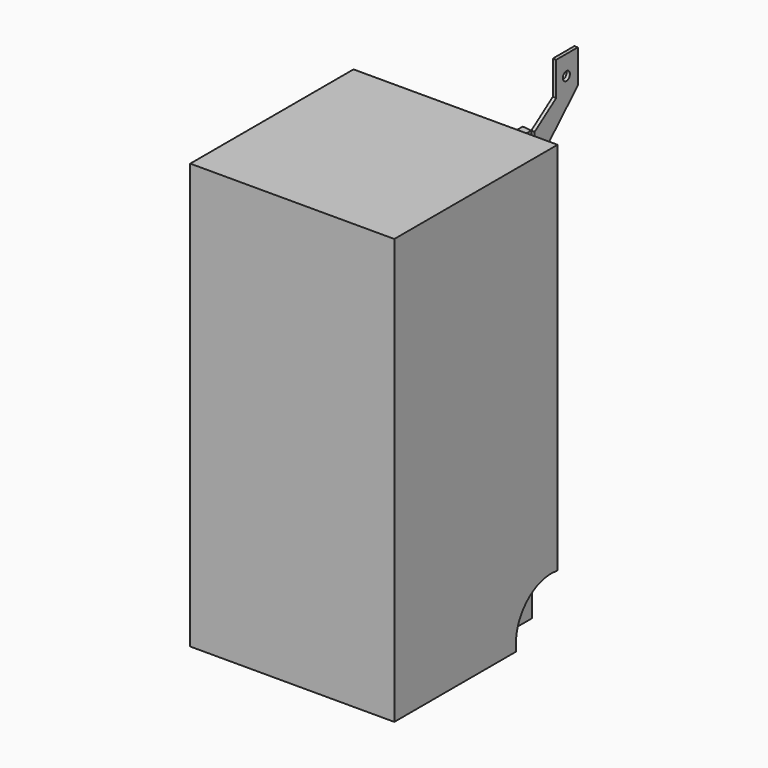
from build123d import *

# Parameters (mm, degrees)
F0_W      = 120
F0_H      = 120
F1_DEPTH  = 250
F4_DEPTH  = 15
F5_DEPTH  = 15
F6_R      = 5
F7_DEPTH  = 90
F11_DEPTH = 10
F12_R     = 2.5839894192
F13_DEPTH = 2


# Not quite as in the source:
# - the program builds the solid bodies; features that only make, move or delete a surface that nothing else refers to are left out


with BuildPart() as f1:
    # F0 (on Top) → F1 (new body)
    with BuildSketch(Plane.XY):
        with Locations((-36.543828845, 41.7243348807)):
            Rectangle(F0_W, F0_H)
    extrude(amount=F1_DEPTH)

    # F3 (on face) → F4 (cut)
    with BuildSketch(Plane(origin=(-96.543828845, 0, 0), x_dir=(0, -1, 0), z_dir=(-1, 0, 0))):
        with BuildLine():
            Line((-101.7243348807, 0), (-71.6849491, 0))
            ThreePointArc((-71.6849491, 0), (-78.6384158471, 23.222277743), (-101.7243348807, 30.6158713042))
            Line((-101.7243348807, 30.6158713042), (-101.7243348807, 0))
        make_face()
    extrude(amount=-F4_DEPTH, mode=Mode.SUBTRACT)

    # F2 (on face) → F5 (cut)
    with BuildSketch(Plane.YZ.offset(23.456171155)):
        with BuildLine():
            Line((101.7243348807, 0), (101.7243348807, 29.543299228))
            ThreePointArc((101.7243348807, 29.543299228), (78.9226920916, 22.6021851134), (71.3572967199, 0))
            Line((71.3572967199, 0), (101.7243348807, 0))
        make_face()
    extrude(amount=-F5_DEPTH, mode=Mode.SUBTRACT)

    # F6 (on face) → F7 (cut)
    with BuildSketch(Plane.YZ.offset(8.456171155)):
        with Locations((89.8642912507, 12.767852284)):
            Circle(F6_R)
    extrude(amount=-F7_DEPTH, mode=Mode.SUBTRACT)

    # F10 (on face) → F11 (join)
    with BuildSketch(Plane(origin=(0, 101.7243348807, 0), x_dir=(-1, 0, 0), z_dir=(0, 1, 0))):
        Polygon((5.0153527409, 246.1044043303), (0, 245.6637322903), (0, 225.8335798979), (5.0153527409, 225.8335798979), align=None)
    extrude(amount=F11_DEPTH)


with BuildPart() as f13:
    # F12 (on face) → F13 (new body)
    with BuildSketch(Plane.YZ):
        Polygon((111.7243348807, 245.6637322903), (111.7243348807, 225.8335798979), (143.3906257153, 256.6804885864), (143.3906257153, 276.5106260777), (127.5265067816, 276.5106260777), (127.5265067816, 256.6804885864), align=None)
        with Locations((135.017901659, 265.0532126427)):
            Circle(F12_R, mode=Mode.SUBTRACT)
    extrude(amount=F13_DEPTH)


solid = Compound([f1.part, f13.part])
